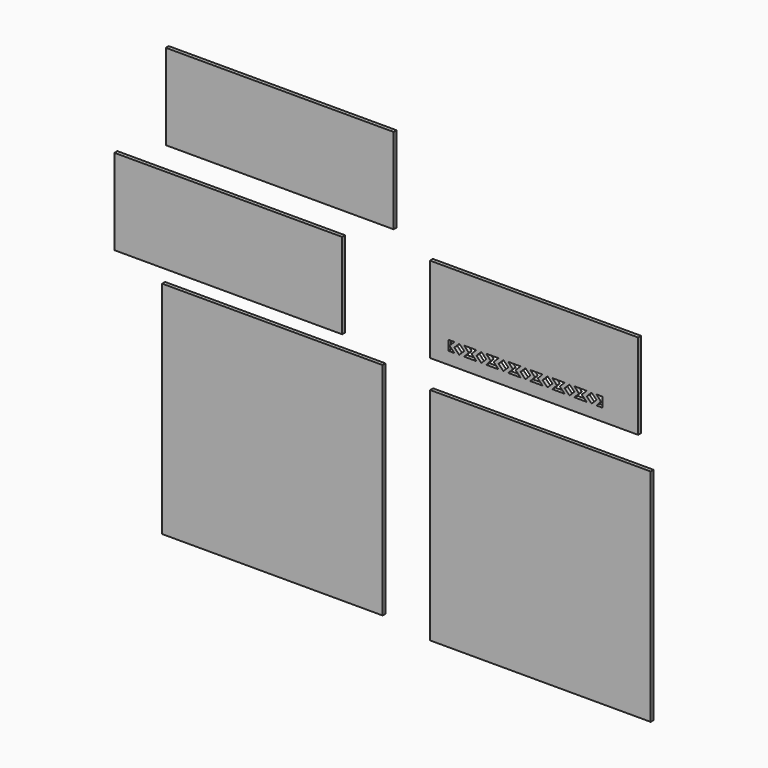
from build123d import *

# Parameters (mm, degrees)
F0_W      = 170
F0_H      = 70
F1_DEPTH  = 3
F3_DEPTH  = 25
F4_W      = 186
F4_H      = 70
F5_DEPTH  = 3
F6_W      = 180
F6_H      = 180
F7_DEPTH  = 3
F8_W      = 186
F8_H      = 70
F9_DEPTH  = 3
F10_W     = 180
F10_H     = 180
F11_DEPTH = 3


# Not quite as in the source:
# - a feature names something its author has since deleted; it is built from what else it names


with BuildPart() as f1:
    # F0 (on Front) → F1 (new body)
    with BuildSketch(Plane.XZ):
        with Locations((27.7395422168, 50.3261041269)):
            Rectangle(F0_W, F0_H)
    extrude(amount=F1_DEPTH)

    # F2 (on face) → F3 (cut)
    with BuildSketch(Plane.XZ.offset(3)):
        Polygon((-42.2604577832, 33.3604037393), (-42.2604577832, 25.3604037393), (-37.2604577832, 25.3604037393), (-41.2604577832, 29.3604037393), (-37.2604577832, 33.3604037393), align=None)
        Polygon((-37.2604524818, 29.366916148), (-33.2604577832, 25.3604037393), (-29.2604630847, 29.366916148), (-33.2604577832, 33.3604037393), align=None)
        Polygon((-25.5732325301, 29.3604037393), (-29.2604577832, 25.3604037393), (-24.2604577832, 25.3604037393), (-24.2604577832, 33.3604037393), (-29.2604577832, 33.3604037393), align=None)
        Polygon((-24.2604577832, 33.3604037393), (-24.2604577832, 25.3604037393), (-19.2604577832, 25.3604037393), (-23.2604577832, 29.3604037393), (-19.2604577832, 33.3604037393), align=None)
        Polygon((-11.2604630847, 29.366916148), (-15.2604577832, 33.3604037393), (-19.2604524818, 29.366916148), (-15.2604577832, 25.3604037393), align=None)
        Polygon((-7.5732325301, 29.3604037393), (-11.2604577832, 25.3604037393), (-6.2604577832, 25.3604037393), (-6.2604577832, 33.3604037393), (-11.2604577832, 33.3604037393), align=None)
        Polygon((-6.2604577832, 33.3604037393), (-6.2604577832, 25.3604037393), (-1.2604577832, 25.3604037393), (-5.2604577832, 29.3604037393), (-1.2604577832, 33.3604037393), align=None)
        Polygon((6.7395369153, 29.366916148), (2.7395422168, 33.3604037393), (-1.2604524818, 29.366916148), (2.7395422168, 25.3604037393), align=None)
        Polygon((10.4267674699, 29.3604037393), (6.7395422168, 25.3604037393), (11.7395422168, 25.3604037393), (11.7395422168, 33.3604037393), (6.7395422168, 33.3604037393), align=None)
        Polygon((11.7395422168, 33.3604037393), (11.7395422168, 25.3604037393), (16.7395422168, 25.3604037393), (12.7395422168, 29.3604037393), (16.7395422168, 33.3604037393), align=None)
        Polygon((24.7395369153, 29.366916148), (20.7395422168, 33.3604037393), (16.7395475182, 29.366916148), (20.7395422168, 25.3604037393), align=None)
        Polygon((28.4267674699, 29.3604037393), (24.7395422168, 25.3604037393), (29.7395422168, 25.3604037393), (29.7395422168, 33.3604037393), (24.7395422168, 33.3604037393), align=None)
        Polygon((29.7395422168, 33.3604037393), (29.7395422168, 25.3604037393), (34.7395422168, 25.3604037393), (30.7395422168, 29.3604037393), (34.7395422168, 33.3604037393), align=None)
        Polygon((42.7395369153, 29.366916148), (38.7395422168, 33.3604037393), (34.7395475182, 29.366916148), (38.7395422168, 25.3604037393), align=None)
        Polygon((46.4267674699, 29.3604037393), (42.7395422168, 25.3604037393), (47.7395422168, 25.3604037393), (47.7395422168, 33.3604037393), (42.7395422168, 33.3604037393), align=None)
        Polygon((47.7395422168, 33.3604037393), (47.7395422168, 25.3604037393), (52.7395422168, 25.3604037393), (48.7395422168, 29.3604037393), (52.7395422168, 33.3604037393), align=None)
        Polygon((60.7395369153, 29.366916148), (56.7395422168, 33.3604037393), (52.7395475182, 29.366916148), (56.7395422168, 25.3604037393), align=None)
        Polygon((64.4267674699, 29.3604037393), (60.7395422168, 25.3604037393), (65.7395422168, 25.3604037393), (65.7395422168, 33.3604037393), (60.7395422168, 33.3604037393), align=None)
        Polygon((65.7395422168, 33.3604037393), (65.7395422168, 25.3604037393), (70.7395422168, 25.3604037393), (66.7395422168, 29.3604037393), (70.7395422168, 33.3604037393), align=None)
        Polygon((78.7395369153, 29.366916148), (74.7395422168, 33.3604037393), (70.7395475182, 29.366916148), (74.7395422168, 25.3604037393), align=None)
        Polygon((82.4267674699, 29.3604037393), (78.7395422168, 25.3604037393), (83.7395422168, 25.3604037393), (83.7395422168, 33.3604037393), (78.7395422168, 33.3604037393), align=None)
    extrude(amount=-F3_DEPTH, mode=Mode.SUBTRACT)


with BuildPart() as f5:
    # F4 (on Front) → F5 (new body)
    with BuildSketch(Plane.XZ):
        with Locations((-221.8526970997, 44.0200128766)):
            Rectangle(F4_W, F4_H)
    extrude(amount=F5_DEPTH)


with BuildPart() as f7:
    # F6 (on Front) → F7 (new body)
    with BuildSketch(Plane.XZ):
        with Locations((33.0046193302, -97.6369565725)):
            Rectangle(F6_W, F6_H)
    extrude(amount=F7_DEPTH)


with BuildPart() as f9:
    # F8 (on Front) → F9 (new body)
    with BuildSketch(Plane.XZ):
        with Locations((-179.8553494937, 133.1439353526)):
            Rectangle(F8_W, F8_H)
    extrude(amount=F9_DEPTH)


with BuildPart() as f11:
    # F10 (on Front) → F11 (new body)
    with BuildSketch(Plane.XZ):
        with Locations((-185.8420636411, -92.3306977749)):
            Rectangle(F10_W, F10_H)
    extrude(amount=F11_DEPTH)


solid = Compound([f1.part, f5.part, f7.part, f9.part, f11.part])
